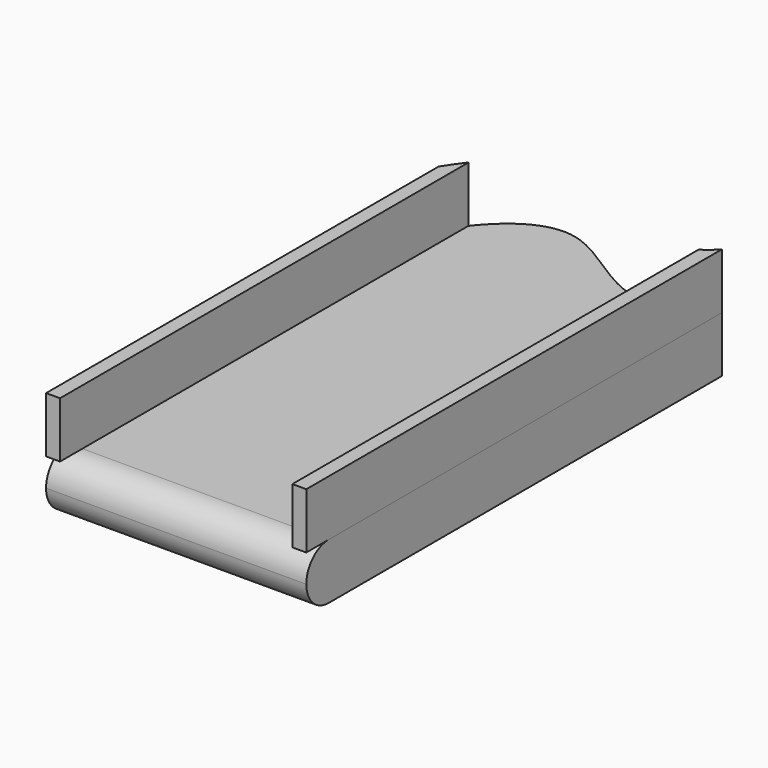
from build123d import *

# Parameters (mm, degrees)
F1_DEPTH = 3657.6
F0_W     = 38.1
F0_H     = 152.4
F2_DEPTH = 3657.6
F3_R     = 76.19999
F5_DEPTH = 457.2


# Not quite as in the source:
# - a fillet or chamfer is up to 0.001 mm smaller than in the source, because OpenCascade refuses the exact size


with BuildPart() as f1:
    # F0 (on Front) → F1 (new body)
    with BuildSketch(Plane.XZ):
        Polygon((355.6, -228.6), (355.6, -76.2), (317.5, -76.2), (-317.5, -76.2), (-355.6, -76.2), (-355.6, -228.6), align=None)
    extrude(amount=-F1_DEPTH)

    # F3 (radius 76.2 in the source; OpenCascade refuses exactly that, so slightly less here)
    f3_edges = [f1.edges().sort_by_distance(p)[0] for p in [
        (0, 0, -76.2),
        (0, 0, -228.6),
        (0, 3657.6, -76.2),
        (0, 3657.6, -228.6),
    ]]
    fillet(f3_edges, radius=F3_R)


with BuildPart() as f2:
    # F0 (on Front) → F2 (new body)
    with BuildSketch(Plane.XZ):
        with Locations((-336.55, 0)):
            Rectangle(F0_W, F0_H)
    extrude(amount=-F2_DEPTH)


with BuildPart() as f2b:
    # F0 (on Front) → F2, piece 2 (new body)
    with BuildSketch(Plane.XZ):
        with Locations((336.55, 0)):
            Rectangle(F0_W, F0_H)
    extrude(amount=-F2_DEPTH)


with BuildPart() as f5_tool:
    # F4 (on face) → F5 (new body)
    with BuildSketch(Plane.XY.offset(76.2)):
        with BuildLine():
            add(Edge.make_bspline(
                [(-355.6, 1340.7233953476), (-915.2366441797, 2359.9510577055), (-1874.2710818809, 3810.9319191607), (44.2691580348, 3688.5723981757), (1019.2784863169, 3988.9601565781), (622.7710571708, 2551.7090574544), (355.6, 1420.0000762939)],
                knots=[0, 0, 0, 0, 0.3063254336, 0.5332153522, 0.6939292156, 1, 1, 1, 1], degree=3))
            Line((-355.6, 1340.7233953476), (-355.6, 3657.6))
            Line((-355.6, 3657.6), (-317.5, 3657.6))
            Line((-317.5, 3657.6), (-317.5, 1395.5652334485))
            add(Edge.make_bspline(
                [(-317.5, 1395.5652334485), (-258.9308915713, 1469.3529332863), (-105.9839814864, 1560.950588612), (119.3033990895, 1321.8331668454), (301.4968463301, 1359.961763396), (355.6, 1420.0000762939)],
                knots=[0.0633807199, 0.0633807199, 0.0633807199, 0.0633807199, 0.3440050043, 0.6929232049, 1, 1, 1, 1], degree=3))
        make_face()
        with BuildLine():
            Line((-355.6, 3657.6), (-355.6, 1340.7233953476))
            add(Edge.make_bspline(
                [(-355.6, 1340.7233953476), (-343.4662540536, 1360.5532417767), (-330.7281932248, 1378.8998277892), (-317.5, 1395.5652334485)],
                knots=[0, 0, 0, 0, 0.0633807199, 0.0633807199, 0.0633807199, 0.0633807199], degree=3))
            Line((-317.5, 1395.5652334485), (-317.5, 3657.6))
            Line((-317.5, 3657.6), (-355.6, 3657.6))
        make_face()
    extrude(amount=-F5_DEPTH)


with BuildPart() as f1_1:
    add(f1.part)

    # F5: cut by f5_tool
    add(f5_tool.part, mode=Mode.SUBTRACT)


with BuildPart() as f2_1:
    add(f2.part)

    # F5: cut by f5_tool
    add(f5_tool.part, mode=Mode.SUBTRACT)


with BuildPart() as f2b_1:
    add(f2b.part)

    # F5: cut by f5_tool
    add(f5_tool.part, mode=Mode.SUBTRACT)


solid = Compound([f1_1.part, f2_1.part, f2b_1.part])
